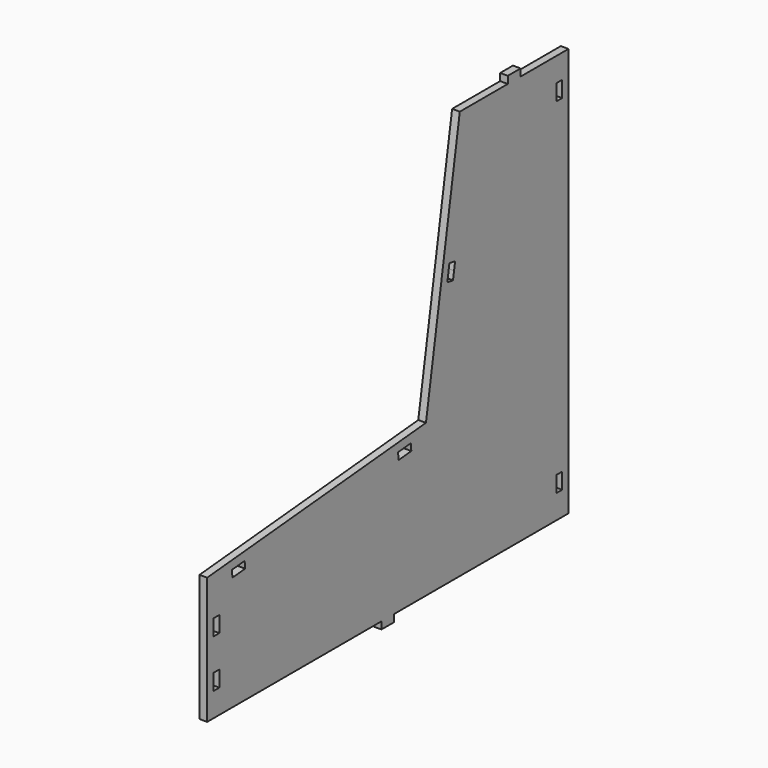
from build123d import *

# Parameters (mm, degrees)
F0_W     = 5
F0_H     = 4.5
F1_DEPTH = 4.8


# Not quite as in the source:
# - a feature names something its author has since deleted; it is built from what else it names


with BuildPart() as f1:
    # F0 (on Right) → F1 (new body)
    with BuildSketch(Plane.YZ):
        Polygon((-531.3379881175, 344.0831357297), (-531.3379881175, 329.0831357297), (-526.3379881175, 329.0831357297), (-526.3379881175, 584.6633606824), (-531.3379881175, 584.6633606824), (-531.3379881175, 569.6633606824), (-531.3379881175, 559.6633606824), (-531.3379881175, 354.0831357297), align=None)
        Polygon((-611.2895517261, 584.6633606824), (-637.7260949769, 424.1829931527), (-639.3722244459, 414.1903303575), (-634.2269114077, 414.6633606824), (-621.0372525622, 494.7298534546), (-620.224537093, 499.6633606824), (-619.4118216237, 504.5968679101), (-606.2221627782, 584.6633606824), align=None)
        Polygon((-803.6983604223, 344.0831357297), (-803.6983604223, 329.0831357297), (-672.5181742699, 329.0831357297), (-672.5181742699, 324.5831357297), (-662.5181742699, 324.5831357297), (-662.5181742699, 329.0831357297), (-531.3379881175, 329.0831357297), (-531.3379881175, 344.0831357297), (-535.8379881175, 344.0831357297), (-535.8379881175, 354.0831357297), (-531.3379881175, 354.0831357297), (-531.3379881175, 559.6633606824), (-535.8379881175, 559.6633606824), (-535.8379881175, 569.6633606824), (-531.3379881175, 569.6633606824), (-531.3379881175, 584.6633606824), (-563.7800754478, 584.6633606824), (-568.7800754478, 584.6633606824), (-573.7800754478, 584.6633606824), (-606.2221627782, 584.6633606824), (-619.4118216237, 504.5968679101), (-614.9716651188, 503.8654239878), (-615.784380588, 498.93191676), (-616.5970960573, 493.9984095323), (-621.0372525622, 494.7298534546), (-634.2269114077, 414.6633606824), (-639.3722244459, 414.1903303575), (-649.1639211663, 413.2901383873), (-659.1219276721, 412.3746568573), (-778.9973858727, 401.3540004817), (-788.9553923784, 400.4385189517), (-803.6983604223, 399.0831357297), (-803.6983604223, 384.0831357297), (-799.1983604223, 384.0831357297), (-799.1983604223, 374.0831357297), (-803.6983604223, 374.0831357297), (-803.6983604223, 354.0831357297), (-799.1983604223, 354.0831357297), (-799.1983604223, 344.0831357297), align=None)
        Polygon((-808.6983604223, 329.0831357297), (-803.6983604223, 329.0831357297), (-803.6983604223, 344.0831357297), (-803.6983604223, 354.0831357297), (-803.6983604223, 374.0831357297), (-803.6983604223, 384.0831357297), (-803.6983604223, 399.0831357297), (-808.6983604223, 399.0831357297), (-808.6983604223, 374.0831357297), (-808.6983604223, 354.0831357297), align=None)
        Polygon((-808.6983604223, 403.4437065252), (-808.6983604223, 399.0831357297), (-803.6983604223, 399.0831357297), (-788.9553923784, 400.4385189517), (-789.3673590669, 404.9196218792), (-779.4093525612, 405.8351034093), (-778.9973858727, 401.3540004817), (-659.1219276721, 412.3746568573), (-659.5338943606, 416.8557597849), (-649.5758878549, 417.7712413149), (-649.1639211663, 413.2901383873), (-639.3722244459, 414.1903303575), (-637.7260949769, 424.1829931527), (-650.0610930658, 423.0489847629), (-808.6983604223, 408.4647918168), align=None)
        with Locations((-566.2800754478, 586.9133606824)):
            Rectangle(F0_W, F0_H)
        with Locations((-571.2800754478, 586.9133606824)):
            Rectangle(F0_W, F0_H)
    extrude(amount=F1_DEPTH)


solid = f1.part
